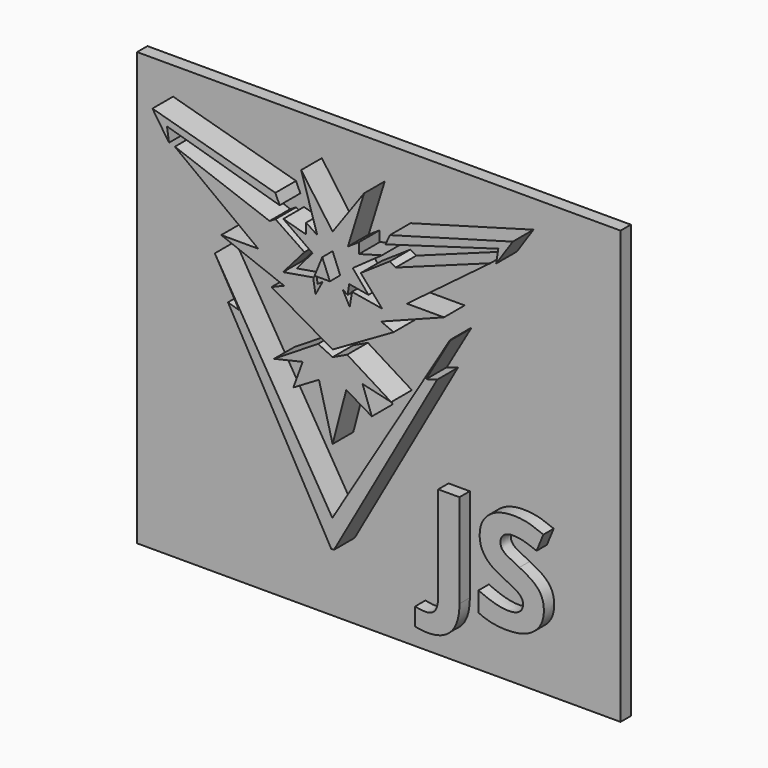
from build123d import *

# Parameters (mm, degrees)
F1_DEPTH     = 7.62
F0_W         = 95
F0_H         = 85
F2_DEPTH     = 2.54
F3_TEXT_SIZE = 27.5921839703
F4_DEPTH     = 2.54
F6_DEPTH     = 2.54


# Not quite as in the source:
# - Text() gives the source's letters only with a copy of the font that has no kerning and outlines rounded to 1/6400 em; it was checked with that copy


with BuildPart() as f1:
    # F0 (on Front) → F1 (new body)
    with BuildSketch(Plane.XZ):
        Polygon((11.9129230734, 36.592964083), (34.0614614543, 43.0456548929), (33.6538197007, 40.3485000134), (36.9149537291, 45.1965518296), (12.7621775027, 38.4707301855), align=None)
    extrude(amount=F1_DEPTH)


with BuildPart() as f1b:
    # F0 (on Front) → F1, piece 2 (new body)
    with BuildSketch(Plane.XZ):
        Polygon((1.2365910225, -13.7706054375), (-21.6437820345, 24.1314768791), (-16.8620757759, 15.8582236618), (-19.0530697121, 16.4965414683), (1.2357736705, -19.5464268327), (1.7781219212, -19.5464268327), (22.0669653039, 16.4965414683), (19.8759713676, 15.8582236618), (24.6576776262, 24.1314768791), (24.5885416961, 24.1776026134), (1.7081686392, -13.7244797032), (1.4697087634, -14.1567725591), align=None)
    extrude(amount=F1_DEPTH)


with BuildPart() as f1c:
    # F0 (on Front) → F1, piece 3 (new body)
    with BuildSketch(Plane.XZ):
        Polygon((1.5069477959, 13.6944502592), (-1.3545840047, 15.056328848), (-10.0100776181, 9.6693439409), (-4.3809800409, 10.9706940129), (-6.1968178488, 5.9468755499), (-1.1730002007, 8.9127449319), (1.5069477959, -1.3326546177), (4.1868957924, 8.9127449319), (9.2107134406, 5.9468755499), (7.3948756326, 10.9706940129), (13.0239732098, 9.6693439409), (4.3684795965, 15.056328848), align=None)
    extrude(amount=F1_DEPTH)


with BuildPart() as f1d:
    # F0 (on Front) → F1, piece 4 (new body)
    with BuildSketch(Plane.XZ):
        Polygon((-9.748281911, 38.4707301855), (-33.9010581374, 45.1965518296), (-30.639924109, 40.3485000134), (-31.0475658625, 43.0456548929), (-8.8990274817, 36.592964083), align=None)
    extrude(amount=F1_DEPTH)


with BuildPart() as f1e:
    # F0 (on Front) → F1, piece 5 (new body)
    with BuildSketch(Plane.XZ):
        Polygon((7.6874790248, 44.0543666482), (1.5069477959, 35.4088284075), (-4.673583433, 44.0543666482), (-1.5064048348, 33.825237304), (-3.6891899072, 35.2804288268), (-3.6891899072, 33.2260429859), (-8.1831589341, 34.4672352076), (-2.447998384, 30.4012615234), (-5.5295773782, 26.7632864416), (-1.7632032977, 27.4052824825), (-1.421541232, 25.4008664631), (-0.4364121996, 26.1212904006), (-1.8488025526, 23.467708379), (-2.3195990361, 26.2496899813), (-8.2234673373, 25.2505746625), (-4.0315873921, 30.0588645041), (-9.7239483148, 33.9108370245), (-10.8795408159, 33.2260429859), (-29.4974129647, 40.0311946869), (-13.1051251665, 27.7048796415), (-20.3810762614, 27.7048796415), (-8.0119594932, 22.9541100562), (-10.4943430051, 21.9269189984), (1.5069477959, 15.0113655254), (13.5082385968, 21.9269189984), (11.0258550849, 22.9541100562), (23.3949718531, 27.7048796415), (16.1190207582, 27.7048796415), (32.5113085564, 40.0311946869), (13.8934364077, 33.2260429859), (12.7378439065, 33.9108370245), (7.0454829838, 30.0588645041), (11.2373629291, 25.2505746625), (5.3334946278, 26.2496899813), (4.8626981443, 23.467708379), (3.4503077914, 26.1212904006), (4.4354368237, 25.4008664631), (4.7770988895, 27.4052824825), (8.5434729699, 26.7632864416), (5.4618939757, 30.4012615234), (11.1970545258, 34.4672352076), (6.7030854989, 33.2260429859), (6.7030854989, 35.2804288268), (4.5203004265, 33.825237304), align=None)
    extrude(amount=F1_DEPTH)

    # F5 (on face) → F6 (join)
    with BuildSketch(Plane.XZ.offset(7.62)):
        Polygon((3, 28.3285770565), (1.5069477959, 32.0338581984), (0, 28.3285770565), align=None)
    extrude(amount=F6_DEPTH)


with BuildPart() as f2:
    # F0 (on Front) → F2 (new body)
    with BuildSketch(Plane.XZ):
        with Locations((6.5272705257, 8.1033739448)):
            Rectangle(F0_W, F0_H)
        Polygon((-16.8620757759, 15.8582236618), (-21.6437820345, 24.1314768791), (1.2365910225, -13.7706054375), (1.4697087634, -14.1567725591), (1.7081686392, -13.7244797032), (24.5885416961, 24.1776026134), (24.6576776262, 24.1314768791), (19.8759713676, 15.8582236618), (22.0669653039, 16.4965414683), (1.7781219212, -19.5464268327), (1.2357736705, -19.5464268327), (-19.0530697121, 16.4965414683), align=None, mode=Mode.SUBTRACT)
        Polygon((-10.0100776181, 9.6693439409), (-1.3545840047, 15.056328848), (1.5069477959, 13.6944502592), (4.3684795965, 15.056328848), (13.0239732098, 9.6693439409), (7.3948756326, 10.9706940129), (9.2107134406, 5.9468755499), (4.1868957924, 8.9127449319), (1.5069477959, -1.3326546177), (-1.1730002007, 8.9127449319), (-6.1968178488, 5.9468755499), (-4.3809800409, 10.9706940129), align=None, mode=Mode.SUBTRACT)
        Polygon((-30.639924109, 40.3485000134), (-33.9010581374, 45.1965518296), (-9.748281911, 38.4707301855), (-8.8990274817, 36.592964083), (-31.0475658625, 43.0456548929), align=None, mode=Mode.SUBTRACT)
        Polygon((-4.673583433, 44.0543666482), (1.5069477959, 35.4088284075), (7.6874790248, 44.0543666482), (4.5203004265, 33.825237304), (6.7030854989, 35.2804288268), (6.7030854989, 33.2260429859), (11.1970545258, 34.4672352076), (5.4618939757, 30.4012615234), (8.5434729699, 26.7632864416), (4.7770988895, 27.4052824825), (4.4354368237, 25.4008664631), (3.4503077914, 26.1212904006), (4.8626981443, 23.467708379), (5.3334946278, 26.2496899813), (11.2373629291, 25.2505746625), (7.0454829838, 30.0588645041), (12.7378439065, 33.9108370245), (13.8934364077, 33.2260429859), (32.5113085564, 40.0311946869), (16.1190207582, 27.7048796415), (23.3949718531, 27.7048796415), (11.0258550849, 22.9541100562), (13.5082385968, 21.9269189984), (1.5069477959, 15.0113655254), (-10.4943430051, 21.9269189984), (-8.0119594932, 22.9541100562), (-20.3810762614, 27.7048796415), (-13.1051251665, 27.7048796415), (-29.4974129647, 40.0311946869), (-10.8795408159, 33.2260429859), (-9.7239483148, 33.9108370245), (-4.0315873921, 30.0588645041), (-8.2234673373, 25.2505746625), (-2.3195990361, 26.2496899813), (-1.8488025526, 23.467708379), (-0.4364121996, 26.1212904006), (-1.421541232, 25.4008664631), (-1.7632032977, 27.4052824825), (-5.5295773782, 26.7632864416), (-2.447998384, 30.4012615234), (-8.1831589341, 34.4672352076), (-3.6891899072, 33.2260429859), (-3.6891899072, 35.2804288268), (-1.5064048348, 33.825237304), align=None, mode=Mode.SUBTRACT)
        Polygon((33.6538197007, 40.3485000134), (34.0614614543, 43.0456548929), (11.9129230734, 36.592964083), (12.7621775027, 38.4707301855), (36.9149537291, 45.1965518296), align=None, mode=Mode.SUBTRACT)
    extrude(amount=F2_DEPTH)

    # F3 (on face) → F4 (join)
    with BuildSketch(Plane.XZ.offset(2.54)):
        with Locations((17.7495479584, -23.8156244159)):
            Text('JS', F3_TEXT_SIZE, font='Open Sans', font_style=FontStyle.BOLD, text_align=(TextAlign.LEFT, TextAlign.BOTTOM))
    extrude(amount=F4_DEPTH)


solid = Compound([f1.part, f1b.part, f1c.part, f1d.part, f1e.part, f2.part])
